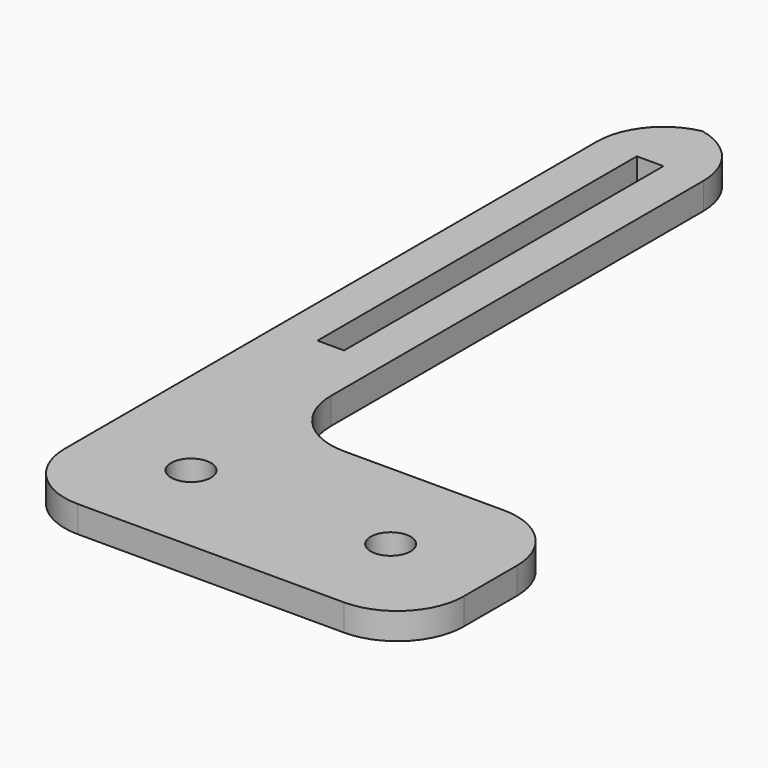
from build123d import *

# Parameters (mm, degrees)
F0_W        = 30
F0_H        = 5
F1_DEPTH    = 2
F2_R        = 5
F3_T1_DEPTH = 27


# Not quite as in the source:
# - a fillet or chamfer that OpenCascade refuses, or shapes differently, is made with other operations: its cross-section is extruded or revolved along the edge and cut away or added
# - a feature names something its author has since deleted; it is built from what else it names


with BuildPart() as f1:
    # F0 (on Top) → F1 (new body)
    with BuildSketch(Plane.XY):
        Polygon((0, 15), (0, 10), (30, 10), (30, 15), (8, 15), (4, 15), align=None)
        with Locations((15, 2.5)):
            Rectangle(F0_W, F0_H)
        with BuildLine():
            Line((0, 7.5), (0, 5))
            Line((0, 5), (30, 5))
            Line((30, 5), (30, 7.5))
            Line((30, 7.5), (24, 7.5))
            ThreePointArc((24, 7.5), (22.5, 6), (21, 7.5))
            Line((21, 7.5), (15, 7.5))
            Line((15, 7.5), (9, 7.5))
            ThreePointArc((9, 7.5), (7.5, 6), (6, 7.5))
            Line((6, 7.5), (0, 7.5))
        make_face()
        with BuildLine():
            Line((0, 10), (0, 7.5))
            Line((0, 7.5), (6, 7.5))
            ThreePointArc((6, 7.5), (7.5, 9), (9, 7.5))
            Line((9, 7.5), (15, 7.5))
            Line((15, 7.5), (21, 7.5))
            ThreePointArc((21, 7.5), (22.5, 9), (24, 7.5))
            Line((24, 7.5), (30, 7.5))
            Line((30, 7.5), (30, 10))
            Line((30, 10), (0, 10))
        make_face()
        Polygon((0, 60), (0, 15), (4, 15), (8, 15), (8, 60), align=None)
        Polygon((5, 25), (4, 25), (3, 25), (3, 55), (5, 55), align=None, mode=Mode.SUBTRACT)
    extrude(amount=F1_DEPTH)

    # F2
    f2_edges = [f1.edges().sort_by_distance(p)[0] for p in [
        (8, 15, 1),
        (30, 15, 1),
        (30, 0, 1),
        (0, 0, 1),
    ]]
    fillet(f2_edges, radius=F2_R)

    # F3: fillet of radius 5 on 2 edges, made by hand

    # F3_s2 → F3_t1 (cut)
    with BuildSketch(Plane.XY.offset(-12.5)):
        with BuildLine():
            ThreePointArc((3, 60), (6.5355339059, 58.5355339059), (8, 55))
            Line((8, 55), (8, 60))
            Line((8, 60), (3, 60))
        make_face()
        with BuildLine():
            ThreePointArc((0, 55), (1.4644660941, 58.5355339059), (5, 60))
            Line((5, 60), (0, 60))
            Line((0, 60), (0, 55))
        make_face()
    extrude(amount=F3_T1_DEPTH, mode=Mode.SUBTRACT)


solid = f1.part
